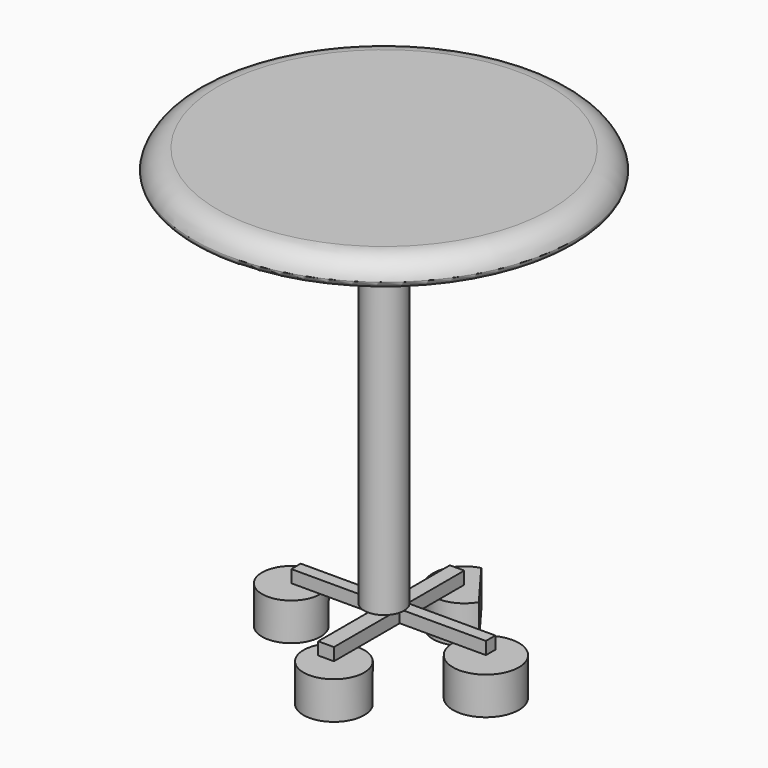
from build123d import *

# Parameters (mm, degrees)
F0_R      = 38.6812763638
F1_DEPTH  = 5.08
F2_R      = 4.0500019282
F3_DEPTH  = 76.2
F4_W      = 3.1792044174
F4_H      = 16.6880693287
F4_W_2    = 18.8102982938
F4_H_2    = 2.3871629965
F4_W_3    = 2.9142722487
F4_H_3    = 14.3064234871
F5_DEPTH  = 2.54
F6_R      = 1.27
F8_R      = 6.6885556935
F8_R_2    = 5.9347433367
F8_R_3    = 6.3640715152
F8_R_4    = 6.1622808629
F9_DEPTH  = 7.62
F11_DEPTH = 7.621


# Not quite as in the source:
# - a fillet or chamfer that OpenCascade refuses, or shapes differently, is made with other operations: its cross-section is extruded or revolved along the edge and cut away or added


with BuildPart() as f1:
    # F0 (on Top) → F1 (new body)
    with BuildSketch(Plane.XY):
        Circle(F0_R)
    extrude(amount=F1_DEPTH)

    # F2 (on face) → F3 (join)
    with BuildSketch(Plane(origin=(0, 0, 0), x_dir=(1, 0, 0), z_dir=(0, 0, -1))):
        Circle(F2_R)
    extrude(amount=F3_DEPTH)

    # F4 (on face) → F5 (join)
    with BuildSketch(Plane(origin=(0, 0, -76.2), x_dir=(1, 0, 0), z_dir=(0, 0, -1))):
        with Locations((1.5896022087, 8.3440346643)):
            Rectangle(F4_W, F4_H)
        Polygon((3.1792044174, 0), (0, 0), (0, -2.3871629965), (2.9142722487, -2.3871629965), (20.6648353487, -2.3871629965), (20.6648353487, 0), align=None)
        with Locations((-9.4051491469, -1.1935814982)):
            Rectangle(F4_W_2, F4_H_2)
        with Locations((1.4571361244, -9.54037474)):
            Rectangle(F4_W_3, F4_H_3)
    extrude(amount=F5_DEPTH)

    # F6
    f6_edges = [f1.edges().sort_by_distance(p)[0] for p in [
        (-38.681276, 0, 0),
    ]]
    fillet(f6_edges, radius=F6_R)

    # F7: fillet of radius 5.08 on 1 edges, made by hand

    # F7_s1 → F7_t2 (revolve, cut)
    with BuildSketch(Plane.XZ):
        with BuildLine():
            ThreePointArc((38.6812763638, 1.27), (36.8734394874, 4.0160926284), (33.7625875141, 5.08))
            Line((33.7625875141, 5.08), (33.7625875141, 5.1816))
            Line((33.7625875141, 5.1816), (38.6812763638, 5.1816))
            Line((38.6812763638, 5.1816), (38.7828763638, 5.08))
            ThreePointArc((38.7828763638, 5.08), (38.7828763638, 3.175), (38.7796501408, 1.2954))
            Line((38.7796501408, 1.2954), (38.6812763638, 1.27))
        make_face()
    revolve(axis=Axis((0, 0, 5.08), (0, 0, 1)), mode=Mode.SUBTRACT)

    # F8 (on face) → F9 (join)
    with BuildSketch(Plane(origin=(0, 0, -78.74), x_dir=(1, 0, 0), z_dir=(0, 0, -1))):
        with Locations((20.6648353487, 0)):
            Circle(F8_R)
        with Locations((-18.8102982938, 0)):
            Circle(F8_R_2)
        with Locations((2.9142722487, -16.6935864836)):
            Circle(F8_R_3)
        with Locations((3.1792044174, 16.6880693287)):
            Circle(F8_R_4)
    extrude(amount=F9_DEPTH)

    # F10 (on face) → F11 (cut, through all)
    with BuildSketch(Plane.XY.offset(-78.74)):
        Polygon((1.4149318504, 22.8785185463), (8.4209625868, 13.5033250881), (25.2221585853, 26.6414508232), (18.2112082839, 35.6629639864), (10.4142271803, 29.6036426698), align=None)
    extrude(amount=-F11_DEPTH, mode=Mode.SUBTRACT)


solid = f1.part
